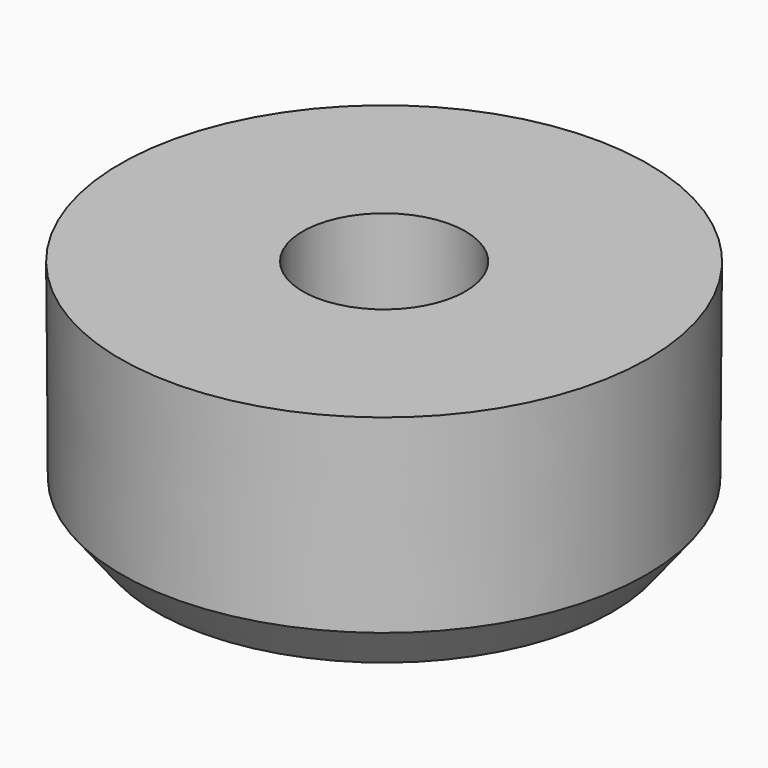
from build123d import *

# Parameters (mm, degrees)
F0_R         = 4.275
F2_R         = 4.925
F4_R         = 4.95
F8_R         = 1.525
F9_DEPTH     = 3.57
F10_R        = 1.3
F11_DEPTH    = 0.83
F13_DEPTH    = 0.46
F14_S5_R     = 1.3
F14_T6_DEPTH = 4


# Not quite as in the source:
# - a fillet or chamfer that OpenCascade refuses, or shapes differently, is made with other operations: its cross-section is extruded or revolved along the edge and cut away or added


with BuildPart() as f6:
    # F0 (on Top) → F6 section 0
    with BuildSketch(Plane.XY):
        Circle(F0_R)
    # F2 (on offset) → F6 section 1
    with BuildSketch(Plane.XY.offset(0.83)):
        Circle(F2_R)
    loft()

    # F2 (on offset) → F7 section 0
    with BuildSketch(Plane.XY.offset(0.83)):
        Circle(F2_R)
    # F4 (on offset) → F7 section 1
    with BuildSketch(Plane.XY.offset(4.4)):
        Circle(F4_R)
    loft()

    # F8 (on face) → F9 (cut, through all)
    with BuildSketch(Plane.XY.offset(4.4)):
        Circle(F8_R)
    extrude(amount=-F9_DEPTH, mode=Mode.SUBTRACT)

    # F10 (on face) → F11 (cut, through all)
    with BuildSketch(Plane(origin=(0, 0, 0), x_dir=(1, 0, 0), z_dir=(0, 0, -1))):
        Circle(F10_R)
    extrude(amount=-F11_DEPTH, mode=Mode.SUBTRACT)

    # F12 (on face) → F13 (cut)
    with BuildSketch(Plane(origin=(0, 0, 0), x_dir=(1, 0, 0), z_dir=(0, 0, -1))):
        Polygon((-0.6, -5), (0, -5), (0.6, -5), (0.6, 0), (0, 0), (-0.6, 0), align=None)
    extrude(amount=-F13_DEPTH, mode=Mode.SUBTRACT)

    # F14: chamfer of 0.5 on 1 edges, made by hand


with BuildPart() as f14_tool2:
    # F14_s3 → F14_t4 (revolve)
    with BuildSketch(Plane.XZ):
        Polygon((1.525, 1.33), (1.025, 0.83), (1.525, 0.83), align=None)
    revolve(axis=Axis((0, 0, 0.83), (0, 0, 1)))

    # F14_s5 → F14_t6 (cut, symmetric)
    with BuildSketch(Plane.XY.offset(1.1)):
        Circle(F14_S5_R)
    extrude(amount=F14_T6_DEPTH, both=True, mode=Mode.SUBTRACT)


with BuildPart() as f6_1:
    add(f6.part)

    # F14_t1: union F14_tool2
    add(f14_tool2.part)


solid = f6_1.part
